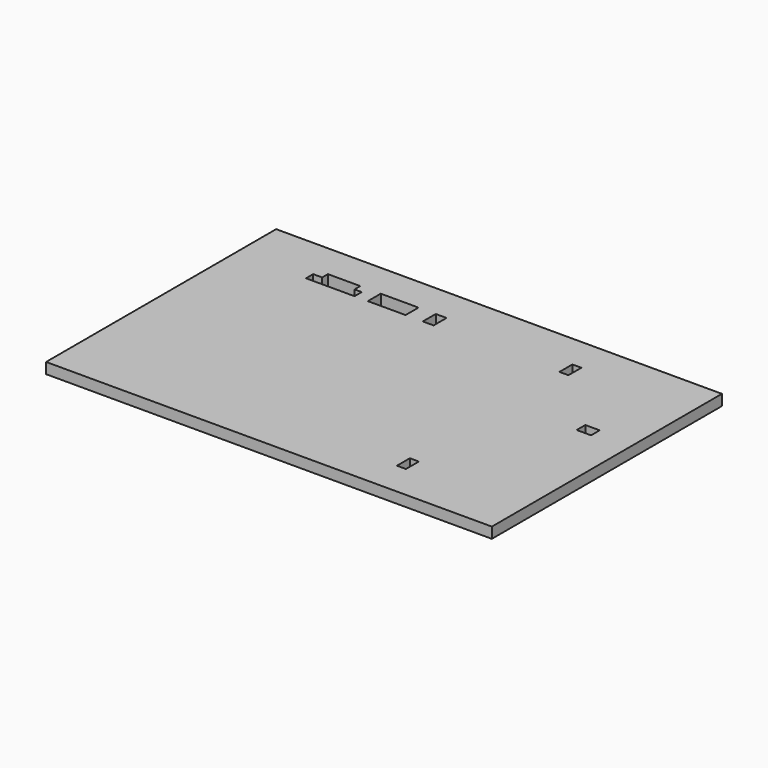
from build123d import *

# Parameters (mm, degrees)
F0_W     = 124
F0_H     = 80
F0_W_2   = 2.5
F0_H_2   = 4.5
F0_W_3   = 10.5
F0_W_4   = 3
F0_W_5   = 4
F0_H_3   = 3
F1_DEPTH = 3


# Not quite as in the source:
# - a feature names something its author has since deleted; it is built from what else it names


with BuildPart() as f1:
    # F0 (on Top) → F1 (new body)
    with BuildSketch(Plane.XY):
        with Locations((-6.0411174464, 30)):
            Rectangle(F0_W, F0_H)
        with Locations((23.2088825536, 1.75)):
            Rectangle(F0_W_2, F0_H_2, mode=Mode.SUBTRACT)
        Polygon((-35.0411174464, 58.5), (-35.0411174464, 56), (-48.5411174464, 56), (-48.5411174464, 58.5), (-46.0411174464, 58.5), (-46.0411174464, 60.5), (-37.0411174464, 60.5), (-37.0411174464, 58.5), align=None, mode=Mode.SUBTRACT)
        with Locations((-26.0911174464, 58.25)):
            Rectangle(F0_W_3, F0_H_2, mode=Mode.SUBTRACT)
        with Locations((-14.5411174464, 58.25)):
            Rectangle(F0_W_4, F0_H_2, mode=Mode.SUBTRACT)
        with Locations((43.9588825536, 38.5)):
            Rectangle(F0_W_5, F0_H_3, mode=Mode.SUBTRACT)
        with Locations((23.2088825536, 58.25)):
            Rectangle(F0_W_2, F0_H_2, mode=Mode.SUBTRACT)
    extrude(amount=F1_DEPTH)


solid = f1.part
